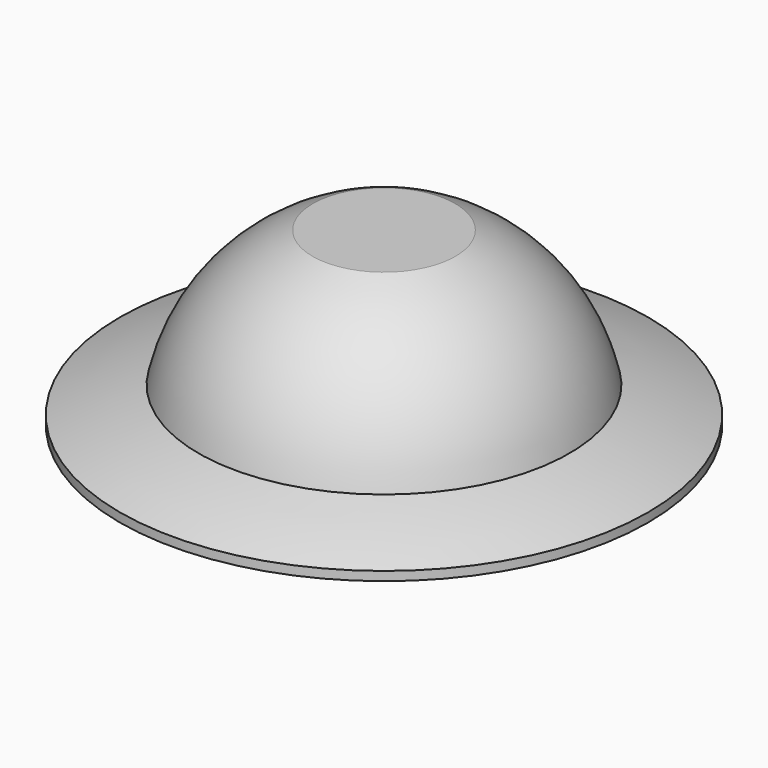
from build123d import *


# Not quite as in the source:
# - ends of sketch curves that miss each other by under 0.0002 mm in the source are joined


with BuildPart() as f1:
    # F0 (on Front) → F1 (revolve)
    with BuildSketch(Plane.XZ):
        with BuildLine():
            ThreePointArc((-23.500000147, -8.2544046337), (-11.967267322, -4.859773912), (0, -3.714367))
            Line((0, -3.714367), (0, 7.013509))
            Line((0, 7.013509), (-6.35, 7.013509))
            ThreePointArc((-6.35, 7.013509), (-12.9335526331, 2.2146110343), (-16.5000003334, -5.1102123602))
            ThreePointArc((-16.5000003334, -5.1102123602), (-20.0343158619, -6.1798378506), (-23.500000147, -7.4544046337))
            Line((-23.500000147, -7.4544046337), (-23.500000147, -8.2544046337))
        make_face()
    revolve(axis=Axis((0, 0, 1.6569155), (0, 0, 1)))


solid = f1.part
